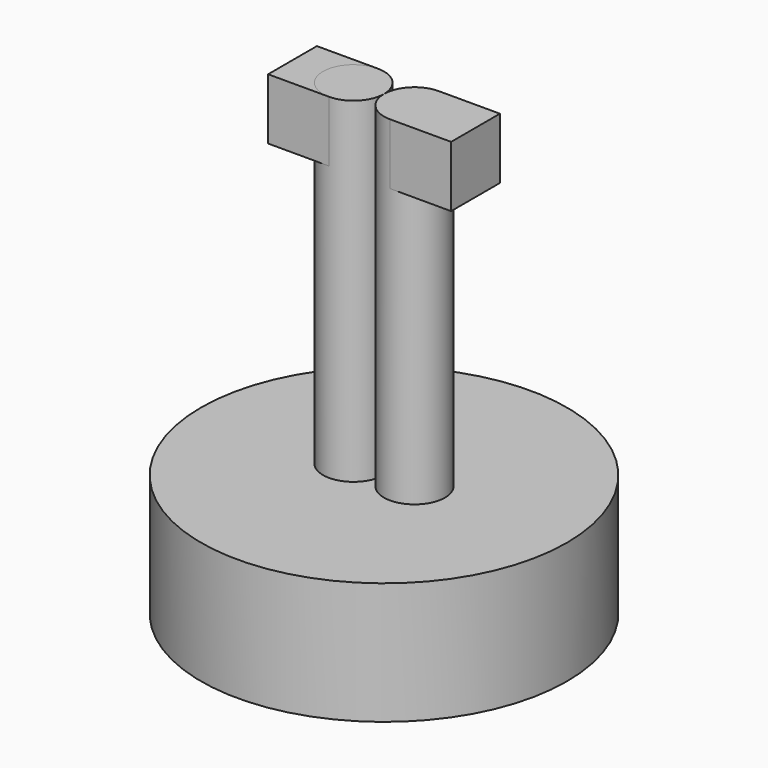
from build123d import *

# Parameters (mm, degrees)
F0_R     = 38.1
F0_R_2   = 6.35
F1_DEPTH = 25.4
F2_DEPTH = 95.25
F4_W     = 12.7
F4_H     = 12.7
F5_DEPTH = 12.7


# Not quite as in the source:
# - a pattern or mirror of a feature is missing from the dataset's text; its kind, count and spacing are read off the source's solid
# - a feature names something its author has since deleted; it is built from what else it names


with BuildPart() as f1:
    # F0 (on Top) → F1 (new body)
    with BuildSketch(Plane.XY):
        Circle(F0_R)
        with Locations((-6.35, 0)):
            Circle(F0_R_2, mode=Mode.SUBTRACT)
        with BuildLine():
            ThreePointArc((12.7, 0), (6.35, -6.35), (0, 0))
            ThreePointArc((0, 0), (6.35, 6.35), (12.7, 0))
        make_face(mode=Mode.SUBTRACT)
        with BuildLine():
            ThreePointArc((12.7, 0), (6.35, 6.35), (0, 0))
            ThreePointArc((0, 0), (6.35, -6.35), (12.7, 0))
        make_face()
        with Locations((-6.35, 0)):
            Circle(F0_R_2)
    extrude(amount=F1_DEPTH)


with BuildPart() as f2:
    # F0 (on Top) → F2 (new body)
    with BuildSketch(Plane.XY):
        with BuildLine():
            ThreePointArc((12.7, 0), (6.35, 6.35), (0, 0))
            ThreePointArc((0, 0), (6.35, -6.35), (12.7, 0))
        make_face()
    extrude(amount=F2_DEPTH)

    # F4 (on offset) → F5 (join)
    with BuildSketch(Plane.YZ.offset(6.35)):
        with Locations((0, 88.9)):
            Rectangle(F4_W, F4_H)
    f5 = extrude(amount=F5_DEPTH)

    # F5_copies: F5 across plane
    add(f5.mirror(Plane(origin=(0, 0, 0), x_dir=(0, 0, -1), z_dir=(-1, 0, 0))))


with BuildPart() as f2b:
    # F0 (on Top) → F2, piece 2 (new body)
    with BuildSketch(Plane.XY):
        with Locations((-6.35, 0)):
            Circle(F0_R_2)
    extrude(amount=F2_DEPTH)


solid = Compound([f1.part, f2.part, f2b.part])
